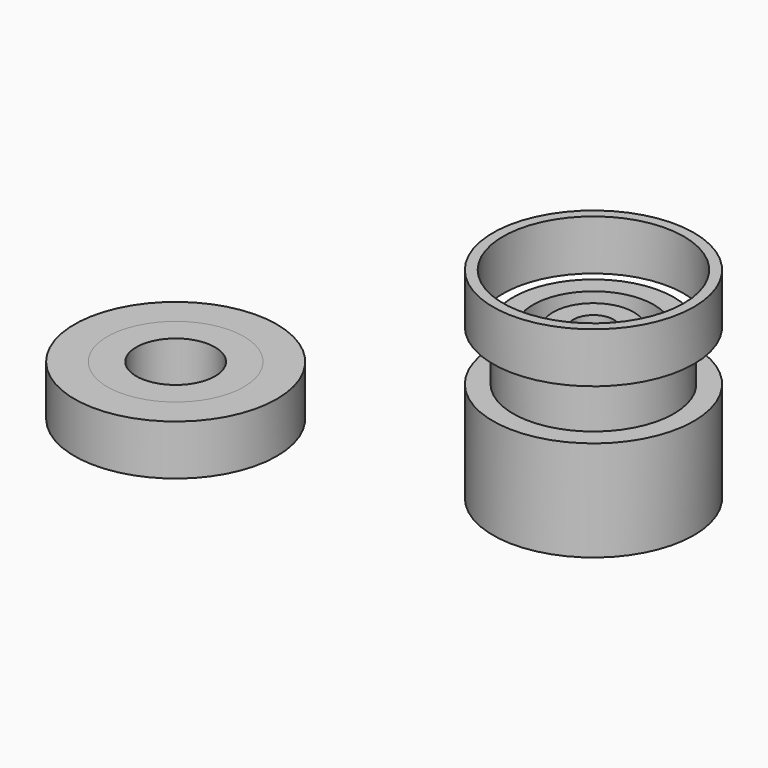
from build123d import *

# Parameters (mm, degrees)
F0_R      = 50
F1_DEPTH  = 50
F2_R      = 40
F2_R_2    = 30
F2_R_3    = 20
F2_R_4    = 10
F3_DEPTH  = 25
F4_R      = 50
F4_R_2    = 45.0000017881
F5_DEPTH  = 25
F6_R      = 50.3499570473
F6_R_2    = 33.9613081037
F7_DEPTH  = 25
F6_R_3    = 19.5827403344
F9_DEPTH  = 25
F10_DEPTH = 25


# Not quite as in the source:
# - a feature of the source that left no trace in its solid (it failed there, or was rolled back) is left out


with BuildPart() as f1:
    # F0 (on Top) → F1 (new body)
    with BuildSketch(Plane.XY):
        Circle(F0_R)
    extrude(amount=-F1_DEPTH)

    # F2 (on Top) → F3 (join)
    with BuildSketch(Plane.XY):
        Circle(F2_R)
        Circle(F2_R_2, mode=Mode.SUBTRACT)
        Circle(F2_R_3)
        Circle(F2_R_4, mode=Mode.SUBTRACT)
    extrude(amount=F3_DEPTH)


with BuildPart() as f5:
    # F4 (on face) → F5 (new body)
    with BuildSketch(Plane.XY.offset(25)):
        Circle(F4_R)
        Circle(F4_R_2, mode=Mode.SUBTRACT)
    extrude(amount=F5_DEPTH)


with BuildPart() as f7:
    # F6 (on Top) → F7 (new body)
    with BuildSketch(Plane.XY):
        with Locations((-108.4925532341, -124.2559552193)):
            Circle(F6_R)
        with Locations((-108.4925532341, -124.2559552193)):
            Circle(F6_R_2, mode=Mode.SUBTRACT)
    extrude(amount=F7_DEPTH)


with BuildPart() as f9:
    # F6 (on Top) → F9 (new body)
    with BuildSketch(Plane.XY):
        with Locations((-108.4925532341, -124.2559552193)):
            Circle(F6_R_2)
        with Locations((-108.4925532341, -124.2559552193)):
            Circle(F6_R_3, mode=Mode.SUBTRACT)
    extrude(amount=F9_DEPTH)


with BuildPart() as f10:
    # F6 (on Top) → F10 (new body)
    with BuildSketch(Plane.XY):
        with Locations((-108.4925532341, -124.2559552193)):
            Circle(F6_R)
        with Locations((-108.4925532341, -124.2559552193)):
            Circle(F6_R_2, mode=Mode.SUBTRACT)
    extrude(amount=F10_DEPTH)


solid = Compound([f1.part, f5.part, f9.part, f10.part])
